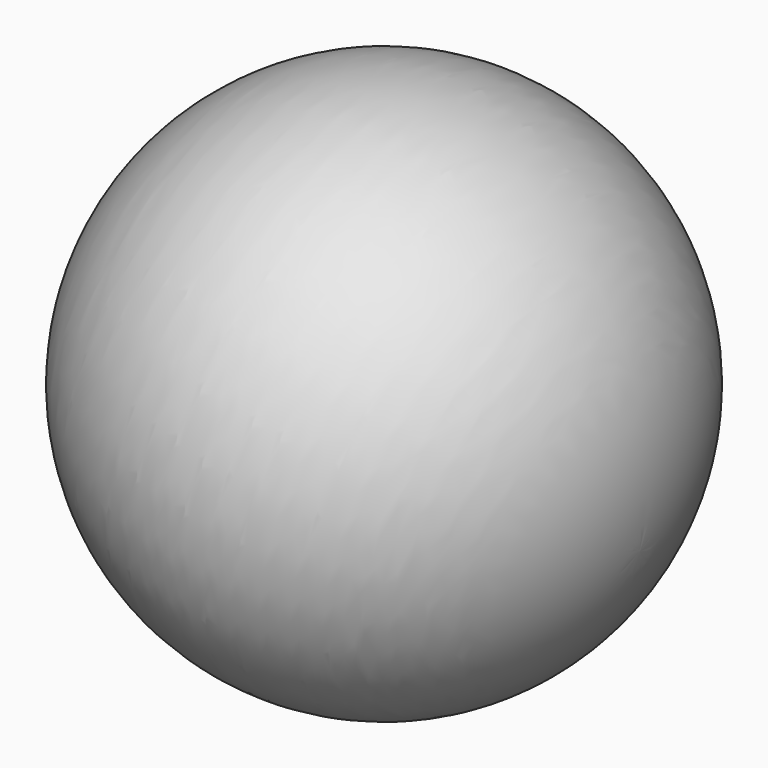
from build123d import *

# Parameters (mm, degrees)
F1_DEPTH = 6.35
F2_R     = 0.508


# Not quite as in the source:
# - a feature of the source that left no trace in its solid (it failed there, or was rolled back) is left out


with BuildPart() as f1:
    # F0 (on Front) → F1 (new body)
    with BuildSketch(Plane.XZ):
        with BuildLine():
            ThreePointArc((-20.6312574446, 56.2981516123), (-20.4548395059, 67.6119681016), (-31.2007516623, 64.0681087971))
            ThreePointArc((-31.2007516623, 64.0681087971), (-41.6528677265, 66.0391478665), (-42.667247355, 55.4512888193))
            Line((-42.667247355, 55.4512888193), (-31.2007516623, 49.0246896703))
            Line((-31.2007516623, 49.0246896703), (-20.6312574446, 56.2981516123))
        make_face()
    extrude(amount=F1_DEPTH)

    # F2
    f2_edges = [f1.edges().sort_by_distance(p)[0] for p in [
        (-20.45484, -6.35, 67.611968),
        (-41.652868, -6.35, 66.039148),
        (-25.916005, -6.35, 52.661421),
        (-36.934, -6.35, 52.237989),
        (-42.667247, -3.175, 55.451289),
        (-31.200752, -3.175, 49.02469),
        (-36.934, 0, 52.237989),
        (-41.652868, 0, 66.039148),
        (-20.45484, 0, 67.611968),
        (-20.631257, -3.175, 56.298152),
        (-25.916005, 0, 52.661421),
    ]]
    fillet(f2_edges, radius=F2_R)


with BuildPart() as f5:
    # F4 (on Front) → F5 (revolve)
    with BuildSketch(Plane.XZ):
        with BuildLine():
            Line((-29.5967943966, 11.3454377279), (15.9822683781, 0))
            ThreePointArc((15.9822683781, 0), (-1.1289024728, 28.4849150576), (-29.5967943966, 11.3454377279))
        make_face()
    revolve(axis=Axis((-6.8072630093, 0, 5.6727188639), (0.9703891035, 0, -0.2415470717)))


solid = f5.part
